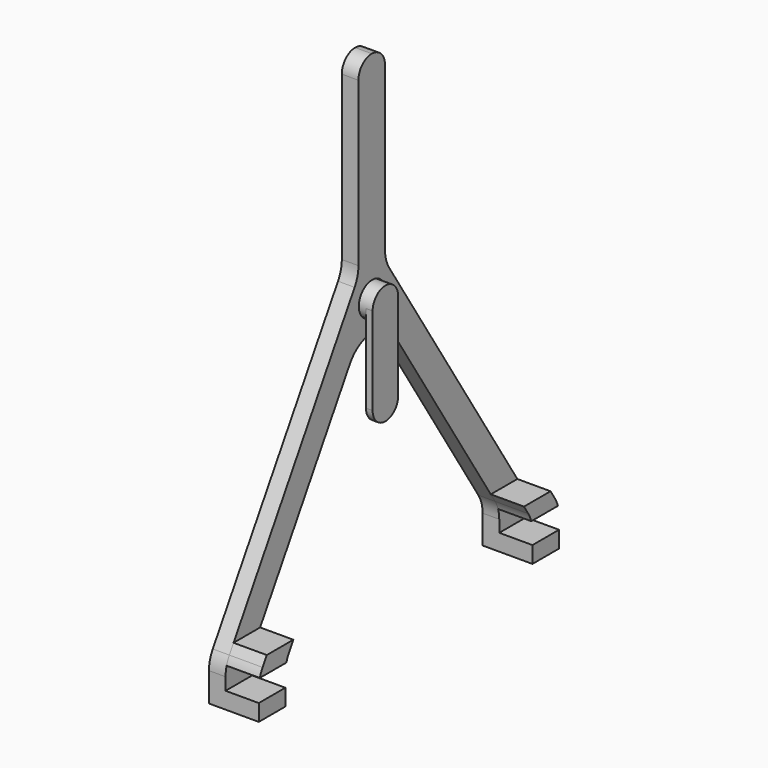
from build123d import *

# Parameters (mm, degrees)
F2_DEPTH  = 5
F3_R      = 10
F4_R      = 4.99999
F5_W      = 10
F5_H      = 5
F6_DEPTH  = 10
F8_DEPTH  = 5
F9_R      = 4.8
F10_DEPTH = 9
F12_DEPTH = 2


# Not quite as in the source:
# - a fillet or chamfer is up to 0.001 mm smaller than in the source, because OpenCascade refuses the exact size


with BuildPart() as f2:
    # F1 (on offset) → F2 (new body)
    with BuildSketch(Plane.YZ.offset(-70)):
        Polygon((-45, 0), (0.145631068, 75), (48, 0), (48, -11.5), (58, -11.5), (58, 0), (5, 83.064516129), (5, 140), (0, 140), (-5, 140), (-5, 83.064516129), (-55, 0), (-55, -11.5), (-45, -11.5), align=None)
    extrude(amount=F2_DEPTH)

    # F3
    f3_edges = [f2.edges().sort_by_distance(p)[0] for p in [
        (-67.5, -55, 0),
        (-67.5, 48, 0),
        (-67.5, 0.145631, 75),
        (-67.5, 5, 83.064516),
        (-67.5, -5, 83.064516),
        (-67.5, 58, 0),
        (-67.5, -45, 0),
    ]]
    fillet(f3_edges, radius=F3_R)

    # F4 (radius 5 in the source; OpenCascade refuses exactly that, so slightly less here)
    f4_edges = [f2.edges().sort_by_distance(p)[0] for p in [
        (-67.5, -5, 140),
        (-67.5, 5, 140),
    ]]
    fillet(f4_edges, radius=F4_R)

    # F5 (on face) → F6 (join)
    with BuildSketch(Plane.YZ.offset(-65)):
        with Locations((-50, -9)):
            Rectangle(F5_W, F5_H)
        with Locations((53, -9)):
            Rectangle(F5_W, F5_H)
        with BuildLine():
            ThreePointArc((-53.5675810852, 2.379663681), (-54.16461993, 1.2236964571), (-54.6065278232, 0))
            Line((-54.6065278232, 0), (-44.6065278232, 0))
            ThreePointArc((-44.6065278232, 0), (-44.16461993, 1.2236964571), (-43.5675810852, 2.379663681))
            Line((-43.5675810852, 2.379663681), (-41.9902912621, 5))
            Line((-41.9902912621, 5), (-51.9902912621, 5))
            Line((-51.9902912621, 5), (-53.5675810852, 2.379663681))
        make_face()
        with BuildLine():
            Line((54.8097087379, 5), (44.8097087379, 5))
            Line((44.8097087379, 5), (46.4301381012, 2.4603739436))
            ThreePointArc((46.4301381012, 2.4603739436), (47.0810932515, 1.2687862909), (47.5646272105, 0))
            Line((47.5646272105, 0), (57.5646272105, 0))
            ThreePointArc((57.5646272105, 0), (57.0810932515, 1.2687862909), (56.4301381012, 2.4603739436))
            Line((56.4301381012, 2.4603739436), (54.8097087379, 5))
        make_face()
    extrude(amount=F6_DEPTH)

    # F7 (on face) → F8 (cut, through all)
    with BuildSketch(Plane.YZ.offset(-70)):
        with BuildLine():
            ThreePointArc((2.8350906603, 70.7849309494), (4.5301092559, 72.5965959517), (5.145631068, 75))
            ThreePointArc((5.145631068, 75), (-2.3147589593, 79.3527555541), (-2.4329612975, 70.7162094574))
            Line((-2.4329612975, 70.7162094574), (0.145631068, 75))
            Line((0.145631068, 75), (2.8350906603, 70.7849309494))
        make_face()
        with BuildLine():
            Line((0.145631068, 75), (-2.4329612975, 70.7162094574))
            ThreePointArc((-2.4329612975, 70.7162094574), (0.2108502857, 70.0004253727), (2.8350906603, 70.7849309494))
            Line((2.8350906603, 70.7849309494), (0.145631068, 75))
        make_face()
    extrude(amount=F8_DEPTH, mode=Mode.SUBTRACT)


with BuildPart() as f10:
    # F9 (on face) → F10 (new body)
    with BuildSketch(Plane.YZ.offset(-70)):
        with Locations((0.145631068, 75)):
            Circle(F9_R)
    extrude(amount=F10_DEPTH)

    # F11 (on face) → F12 (join)
    with BuildSketch(Plane.YZ.offset(-61)):
        with BuildLine():
            Line((4.945631068, 75), (-4.654368932, 75))
            Line((-4.654368932, 75), (-4.654368932, 48.6))
            ThreePointArc((-4.654368932, 48.6), (0.145631068, 53.4), (4.945631068, 48.6))
            Line((4.945631068, 48.6), (4.945631068, 75))
        make_face()
        with BuildLine():
            ThreePointArc((4.945631068, 48.6), (0.145631068, 53.4), (-4.654368932, 48.6))
            Line((-4.654368932, 48.6), (4.945631068, 48.6))
        make_face()
        with BuildLine():
            Line((4.945631068, 48.6), (-4.654368932, 48.6))
            ThreePointArc((-4.654368932, 48.6), (0.145631068, 43.8), (4.945631068, 48.6))
        make_face()
        with BuildLine():
            ThreePointArc((4.945631068, 75), (0.145631068, 79.8), (-4.654368932, 75))
            Line((-4.654368932, 75), (4.945631068, 75))
        make_face()
    extrude(amount=-F12_DEPTH)


solid = Compound([f2.part, f10.part])
